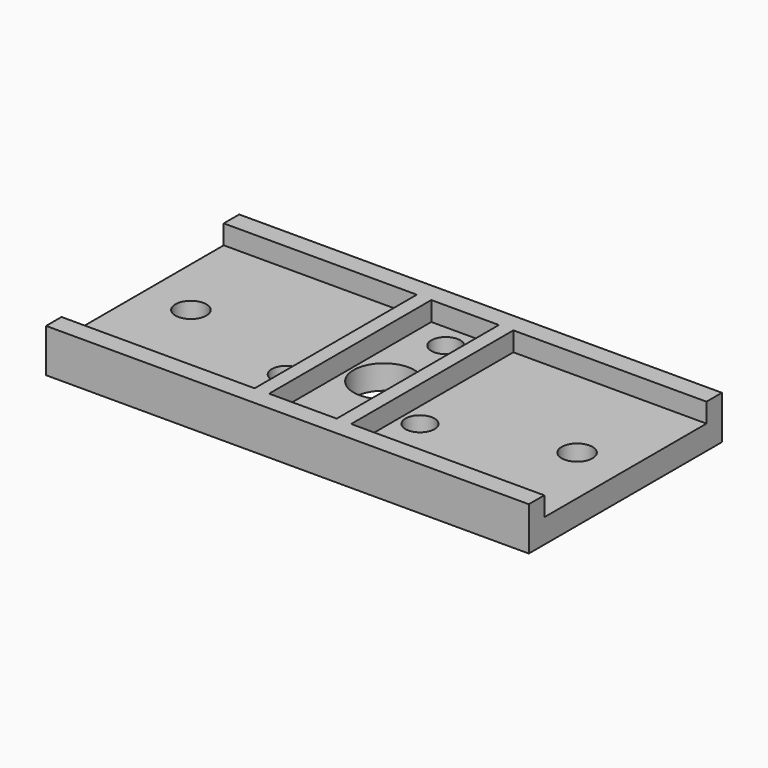
from build123d import *

# Parameters (mm, degrees)
F0_W            = 50
F0_H            = 25
F0_R            = 1.6
F0_R_2          = 3.15
F1_DEPTH        = 2.5
F2_R            = 1.5
F3_DEPTH        = 25
F3_COPIES_COUNT = 3
F4_W            = 1.5
F4_H            = 21
F5_DEPTH        = 2


# Not quite as in the source:
# - a pattern or mirror of a feature is missing from the dataset's text; its kind, count and spacing are read off the source's solid


with BuildPart() as f1:
    # F0 (on Top) → F1 (new body)
    with BuildSketch(Plane.XY):
        Rectangle(F0_W, F0_H)
        with Locations((-20, 0)):
            Circle(F0_R, mode=Mode.SUBTRACT)
        Circle(F0_R_2, mode=Mode.SUBTRACT)
        with Locations((20, 0)):
            Circle(F0_R, mode=Mode.SUBTRACT)
    extrude(amount=F1_DEPTH)

    # F2 (on face) → F3 (cut)
    with BuildSketch(Plane.XY.offset(2.5)):
        with Locations((0, 8)):
            Circle(F2_R)
    f3 = extrude(amount=-F3_DEPTH, mode=Mode.SUBTRACT)

    # F3_copies: F3 ×3 about axis
    f3_copies_axis = Axis((0, 0, 0), (0, 0, 1))
    for i in range(1, F3_COPIES_COUNT):
        add(f3.rotate(f3_copies_axis, i * 360 / F3_COPIES_COUNT), mode=Mode.SUBTRACT)

    # F4 (on face) → F5 (join)
    with BuildSketch(Plane.XY.offset(2.5)):
        Polygon((25, 12.5), (-25, 12.5), (-25, 10.5), (-5, 10.5), (-3.5, 10.5), (3.5, 10.5), (5, 10.5), (25, 10.5), align=None)
        with Locations((-4.25, 0)):
            Rectangle(F4_W, F4_H)
        with Locations((4.25, 0)):
            Rectangle(F4_W, F4_H)
        Polygon((-3.5, -10.5), (-5, -10.5), (-25, -10.5), (-25, -12.5), (25, -12.5), (25, -10.5), (5, -10.5), (3.5, -10.5), align=None)
    extrude(amount=F5_DEPTH)


solid = f1.part
